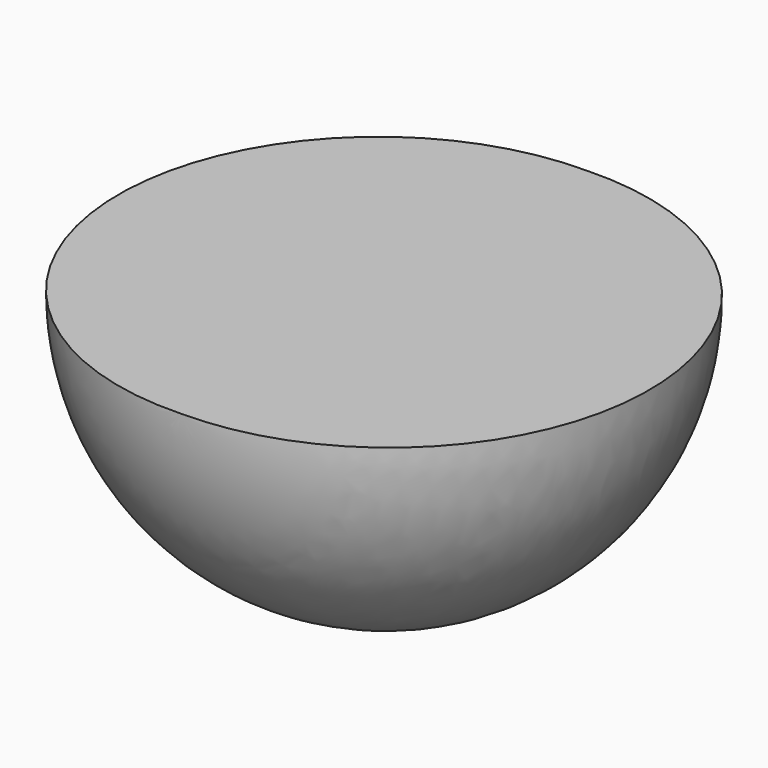
from build123d import *

# Parameters (mm, degrees)
F3_ANGLE = 180


# Not quite as in the source:
# - the program builds the solid bodies; features that only make, move or delete a surface that nothing else refers to are left out


with BuildPart() as f3:
    # F2 (on face) → F3 (revolve)
    with BuildSketch(Plane.XY):
        with BuildLine():
            Line((1.5253506135, -47.4100708961), (0, 46.0746884346))
            ThreePointArc((0, 46.0746884346), (-46.9927618933, -1.4468961616), (1.5253506135, -47.4100708961))
        make_face()
    revolve(axis=Axis((0.7626753068, -0.6676912308, 0), (0.0163143984, -0.9998669113, 0)), revolution_arc=F3_ANGLE)


solid = f3.part
